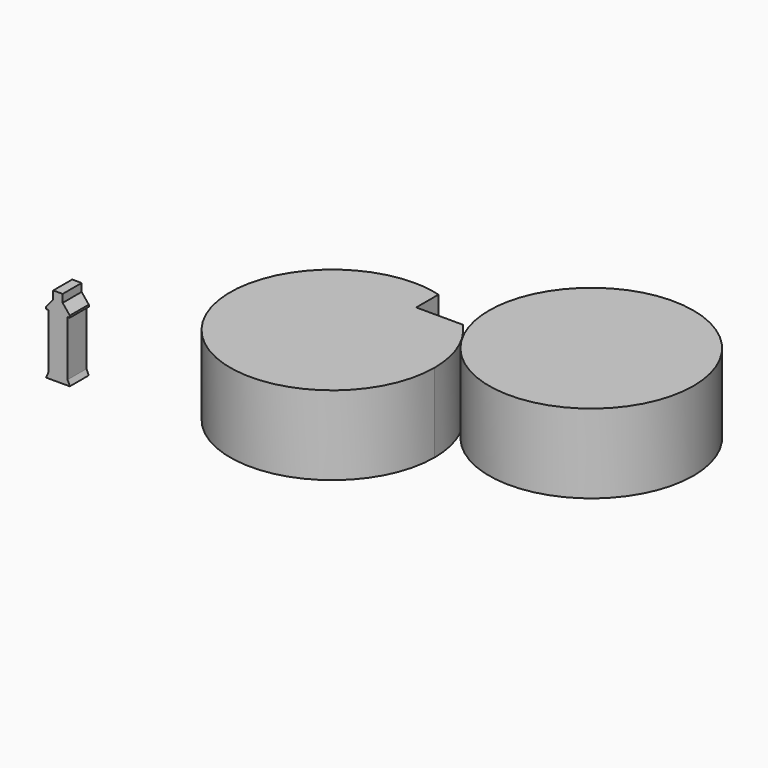
from build123d import *

# Parameters (mm, degrees)
F1_DEPTH = 63.5
F2_W     = 19.05
F2_H     = 19.05
F3_DEPTH = 63.5
F5_DEPTH = 25.4
F6_DEPTH = 25.4


with BuildPart() as f1:
    # F0 (on Top) → F1 (new body)
    with BuildSketch(Plane.XY):
        with BuildLine():
            ThreePointArc((3.706e-07, 82.0754298145), (-58.0360931216, -58.0360928596), (82.0754298145, 0))
            ThreePointArc((82.0754298145, 0), (76.1852973221, 30.5315681088), (59.3603090217, 56.6809482285))
            Line((59.3603090217, 56.6809482285), (21.9643415828, 56.6809482285))
            Line((21.9643415828, 56.6809482285), (21.9643415828, 79.0818808455))
            ThreePointArc((21.9643415828, 79.0818808455), (11.0837003396, 81.3235990719), (3.706e-07, 82.0754298145))
        make_face()
    extrude(amount=F1_DEPTH)


with BuildPart() as f1b:
    # F0 (on Top) → F1, piece 2 (new body)
    with BuildSketch(Plane.XY):
        with BuildLine():
            Line((72.7643415828, 56.6809482285), (64.2149444137, 56.6809482285))
            ThreePointArc((64.2149444137, 56.6809482285), (155.1189122788, 1.0131001695), (224.3384138205, 82.0754298145))
            ThreePointArc((224.3384138205, 82.0754298145), (155.124643919, 163.136850253), (64.2185363282, 107.4809482285))
            Line((64.2185363282, 107.4809482285), (72.7643415828, 107.4809482285))
            Line((72.7643415828, 107.4809482285), (72.7643415828, 56.6809482285))
        make_face()
        with BuildLine():
            ThreePointArc((64.2185363282, 107.4809482285), (60.1875543967, 82.0812331201), (64.2149444137, 56.6809482285))
            Line((64.2149444137, 56.6809482285), (72.7643415828, 56.6809482285))
            Line((72.7643415828, 56.6809482285), (72.7643415828, 107.4809482285))
            Line((72.7643415828, 107.4809482285), (64.2185363282, 107.4809482285))
        make_face()
    extrude(amount=F1_DEPTH)


with BuildPart() as f3:
    # F2 (on Top) → F3 (new body)
    with BuildSketch(Plane.XY):
        with Locations((-166.4411127567, -57.9276421648)):
            Rectangle(F2_W, F2_H)
    extrude(amount=F3_DEPTH)

    # F4 (on face) → F5 (cut)
    with BuildSketch(Plane.XZ.offset(67.4526421648)):
        Polygon((-162.651643157, 57.180352509), (-156.9161127567, 50.0548891723), (-156.9161127567, 63.5), (-162.651643157, 63.5), align=None)
        Polygon((-158.6997658014, 4.1012191214), (-156.9161127567, 0), (-156.9161127567, 48.4922751784), (-158.6997658014, 48.4922751784), align=None)
    extrude(amount=-F5_DEPTH, mode=Mode.SUBTRACT)

    # F4 (on face) → F6 (cut)
    with BuildSketch(Plane.XZ.offset(67.4526421648)):
        Polygon((-170.2305823565, 57.180352509), (-170.2305823565, 63.5), (-175.9661127567, 63.5), (-175.9661127567, 50.0548891723), align=None)
        Polygon((-175.9661127567, 48.4922751784), (-175.9661127567, 0), (-174.182459712, 4.1012191214), (-174.182459712, 48.4922751784), align=None)
    extrude(amount=-F6_DEPTH, mode=Mode.SUBTRACT)


solid = Compound([f1.part, f1b.part, f3.part])
